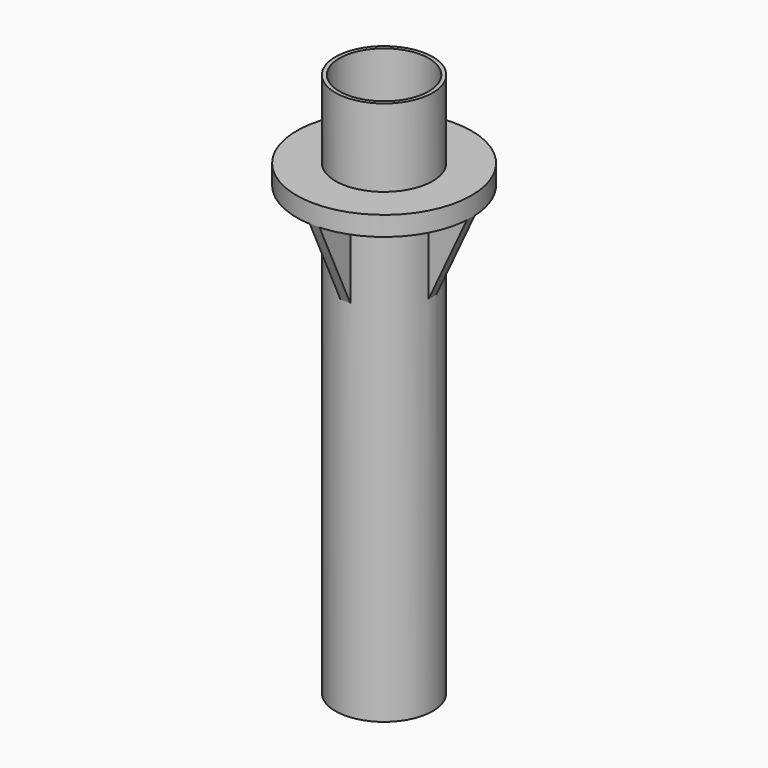
from build123d import *

# Parameters (mm, degrees)
F0_R            = 31.75
F1_DEPTH        = 304.8
F2_R            = 28.575
F3_DEPTH        = 292.1
F4_R            = 57.15
F4_R_2          = 31.75
F5_DEPTH        = 12.7
F7_DEPTH        = 3.175
F7_COPIES_COUNT = 4
F8_R            = 31.75
F9_DEPTH        = 50.8
F10_R           = 29.21
F11_DEPTH       = 87.884


# Not quite as in the source:
# - a pattern or mirror of a feature is missing from the dataset's text; its kind, count and spacing are read off the source's solid


with BuildPart() as f1:
    # F0 (on Top) → F1 (new body)
    with BuildSketch(Plane.XY):
        Circle(F0_R)
    extrude(amount=F1_DEPTH)

    # F2 (on face) → F3 (cut)
    with BuildSketch(Plane.XY.offset(304.8)):
        Circle(F2_R)
    extrude(amount=-F3_DEPTH, mode=Mode.SUBTRACT)

    # F4 (on face) → F5 (join)
    with BuildSketch(Plane.XY.offset(304.8)):
        Circle(F4_R)
        Circle(F4_R_2, mode=Mode.SUBTRACT)
    extrude(amount=-F5_DEPTH)

    # F6 (on Right) → F7 (join, symmetric)
    with BuildSketch(Plane.YZ):
        Polygon((30.9059452266, 236.7404699326), (56.9043979049, 292.3926711082), (30.9059452266, 290.2498841286), align=None)
    f7 = extrude(amount=F7_DEPTH, both=True)

    # F7_copies: F7 ×4 about axis
    f7_copies_axis = Axis((0, 0, 0), (0, 0, 1))
    for i in range(1, F7_COPIES_COUNT):
        add(f7.rotate(f7_copies_axis, i * 360 / F7_COPIES_COUNT))

    # F8 (on face) → F9 (join)
    with BuildSketch(Plane.XY.offset(304.8)):
        Circle(F8_R)
    extrude(amount=F9_DEPTH)

    # F10 (on face) → F11 (cut)
    with BuildSketch(Plane.XY.offset(355.6)):
        Circle(F10_R)
    extrude(amount=-F11_DEPTH, mode=Mode.SUBTRACT)


solid = f1.part
